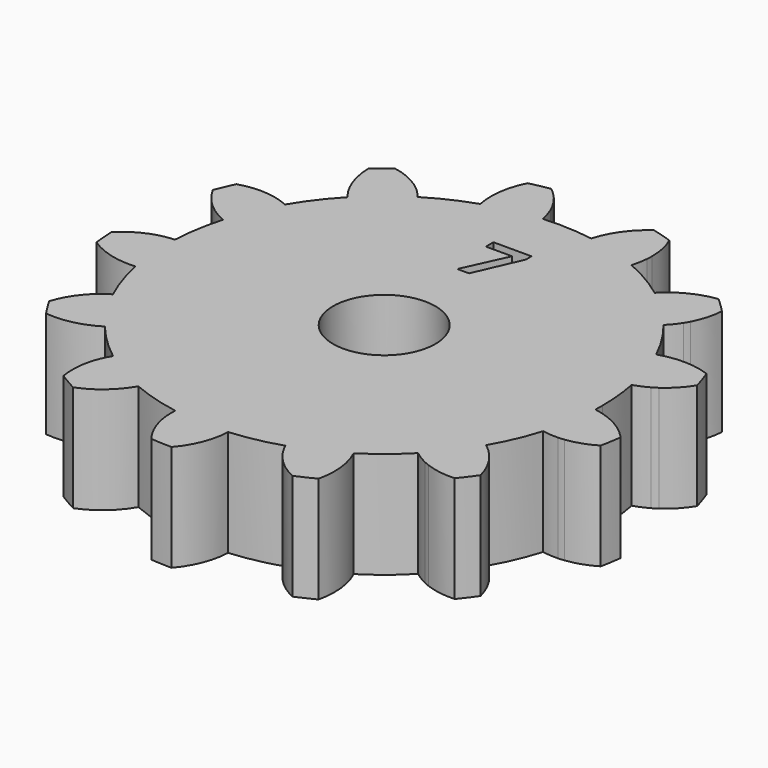
from build123d import *

# Parameters (mm, degrees)
F1_DEPTH     = 10
F2_COUNT     = 13
F3_R         = 4.8125
F4_DEPTH     = 6
F5_R         = 2
F6_DEPTH     = 4
F7_TEXT_SIZE = 6.9895966185
F8_DEPTH     = 2


# Not quite as in the source:
# - Text() gives the source's letters only with a copy of the font that has no kerning and outlines rounded to 1/6400 em; it was checked with that copy


with BuildPart() as f1:
    # F0 (on Top) → F1 (new body)
    with BuildSketch(Plane.XY):
        with BuildLine():
            ThreePointArc((7.9284276206, 23.5955864404), (6.9900144894, 23.8904031242), (6.04068631, 24.1479144628))
            ThreePointArc((6.04068631, 24.1479144628), (4.3213940573, 22.4329291679), (3.263536476, 20.2470477097))
            ThreePointArc((3.263536476, 20.2470477097), (5.7825841651, 19.676263153), (8.2099093234, 18.7933764979))
            ThreePointArc((8.2099093234, 18.7933764979), (8.3945552331, 19.5156155745), (8.498494095, 20.2538026162))
            ThreePointArc((8.498494095, 20.2538026162), (8.5166436171, 20.5392033965), (8.5226970743, 20.825116611))
            ThreePointArc((8.5226970743, 20.825116611), (8.3724590035, 22.2418610533), (7.9284276206, 23.5955864404))
        make_face()
        with BuildLine():
            ThreePointArc((4.0253666655, 14.4585201562), (-1.7454613083, 15.0554452906), (-4.9249243377, 19.9082578735))
            ThreePointArc((-4.9249243377, 19.9082578735), (-12.6410323189, -16.1492387809), (20.5083790508, 0))
            ThreePointArc((20.5083790508, 0), (19.2412101906, 7.0971432063), (15.5962949152, 13.3172518264))
            ThreePointArc((15.5962949152, 13.3172518264), (9.5252611173, 10.9925929993), (4.0253666655, 14.4585201562))
        make_face()
        with BuildLine():
            ThreePointArc((3.263536476, 20.2470477097), (-0.8477895051, 20.4908483047), (-4.9249243377, 19.9082578735))
            ThreePointArc((-4.9249243377, 19.9082578735), (-1.7454613083, 15.0554452906), (4.0253666655, 14.4585201562))
            ThreePointArc((4.0253666655, 14.4585201562), (3.0372062455, 17.2728641577), (3.263536476, 20.2470477097))
        make_face()
        with BuildLine():
            ThreePointArc((4.0253666655, 14.4585201562), (9.5252611173, 10.9925929993), (15.5962949152, 13.3172518264))
            ThreePointArc((15.5962949152, 13.3172518264), (12.2139602675, 16.4746103406), (8.2099093234, 18.7933764979))
            ThreePointArc((8.2099093234, 18.7933764979), (6.6277035692, 16.133569575), (4.0253666655, 14.4585201562))
        make_face()
        with BuildLine():
            ThreePointArc((8.2099093234, 18.7933764979), (5.7825841651, 19.676263153), (3.263536476, 20.2470477097))
            ThreePointArc((3.263536476, 20.2470477097), (3.0372062455, 17.2728641577), (4.0253666655, 14.4585201562))
            ThreePointArc((4.0253666655, 14.4585201562), (6.6277035692, 16.133569575), (8.2099093234, 18.7933764979))
        make_face()
    extrude(amount=F1_DEPTH)

    # F2: F1 ×13 about axis
    f2_axis = Axis((0, 0, 10), (0, 0, 1))


with BuildPart() as f1_1:
    add(f1.part)
    for i in range(1, F2_COUNT):
        add(f1.part.rotate(f2_axis, i * 360 / F2_COUNT))

    # F3 (on face) → F4 (cut)
    with BuildSketch(Plane.XY.offset(10)):
        Circle(F3_R)
    extrude(amount=-F4_DEPTH, mode=Mode.SUBTRACT)

    # F5 (on face) → F6 (join)
    with BuildSketch(Plane(origin=(0, 0, 0), x_dir=(1, 0, 0), z_dir=(0, 0, -1))):
        Circle(F5_R)
    extrude(amount=F6_DEPTH)

    # F7 (on face) → F8 (cut)
    with BuildSketch(Plane.XY.offset(10)):
        with Locations((-2.153794514, 10.3121809661)):
            Text('7', F7_TEXT_SIZE, font='Open Sans', font_style=FontStyle.BOLD, text_align=(TextAlign.LEFT, TextAlign.BOTTOM))
    extrude(amount=-F8_DEPTH, mode=Mode.SUBTRACT)


solid = f1_1.part
